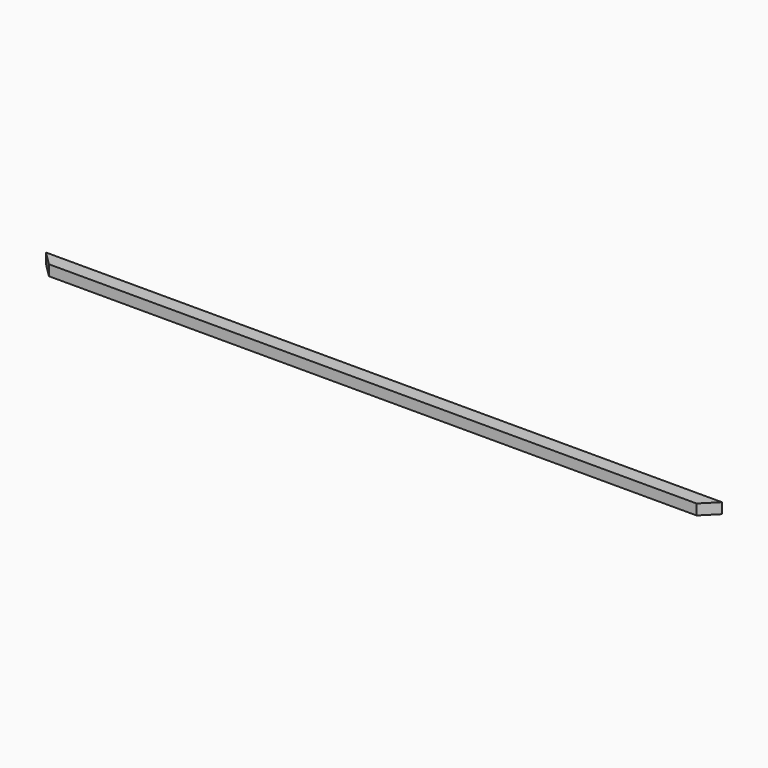
from build123d import *

# Parameters (mm, degrees)
F0_W     = 1219.2
F0_H     = 25.4
F1_DEPTH = 19.05
F2_SIZE  = 25.39999


# Not quite as in the source:
# - a fillet or chamfer is up to 0.001 mm smaller than in the source, because OpenCascade refuses the exact size


with BuildPart() as f1:
    # F0 (on Top) → F1 (new body)
    with BuildSketch(Plane.XY):
        with Locations((188.7929144382, -134.3236717459)):
            Rectangle(F0_W, F0_H)
    extrude(amount=F1_DEPTH)

    # F2 (size 25.4 in the source; OpenCascade refuses exactly that, so slightly less here)
    f2_edges = [f1.edges().sort_by_distance(p)[0] for p in [
        (798.392914, -147.023672, 9.525),
        (-420.807086, -147.023672, 9.525),
    ]]
    chamfer(f2_edges, length=F2_SIZE)


solid = f1.part
